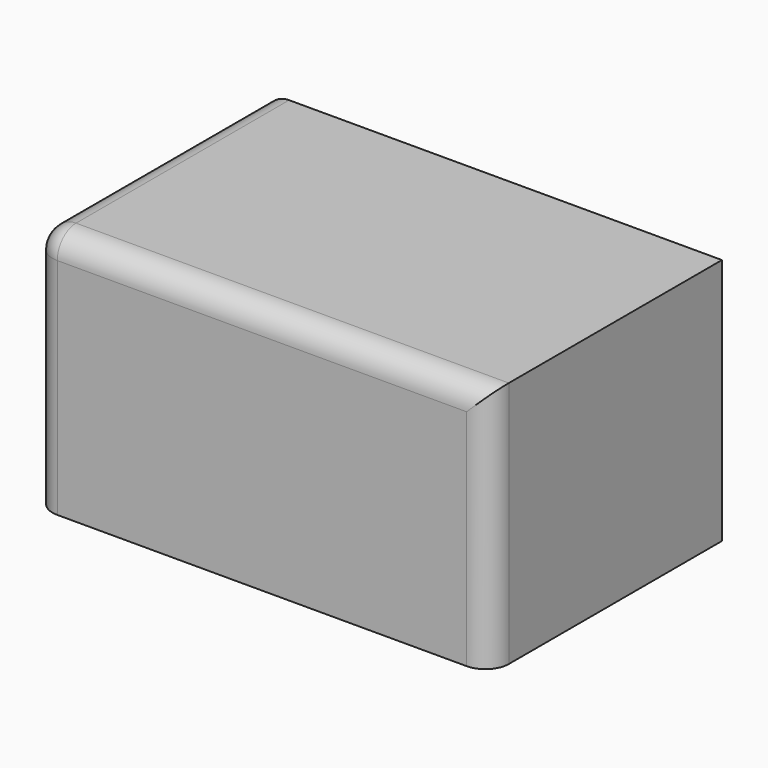
from build123d import *

# Parameters (mm, degrees)
F0_W     = 97.4512062967
F0_H     = 52.8376847506
F1_DEPTH = 61.9
F4_R     = 5


# Not quite as in the source:
# - a feature of the source that left no trace in its solid (it failed there, or was rolled back) is left out


with BuildPart() as f1:
    # F0 (on Front) → F1 (new body)
    with BuildSketch(Plane.XZ):
        with Locations((-12.1814031154, 3.6894287914)):
            Rectangle(F0_W, F0_H)
    extrude(amount=F1_DEPTH)

    # F4
    f4_edges = [f1.edges().sort_by_distance(p)[0] for p in [
        (-60.907006, -30.95, 30.108271),
        (-12.181403, -61.9, 30.108271),
        (-60.907006, -61.9, 3.689429),
        (36.5442, -61.9, 3.689429),
    ]]
    fillet(f4_edges, radius=F4_R)


solid = f1.part
